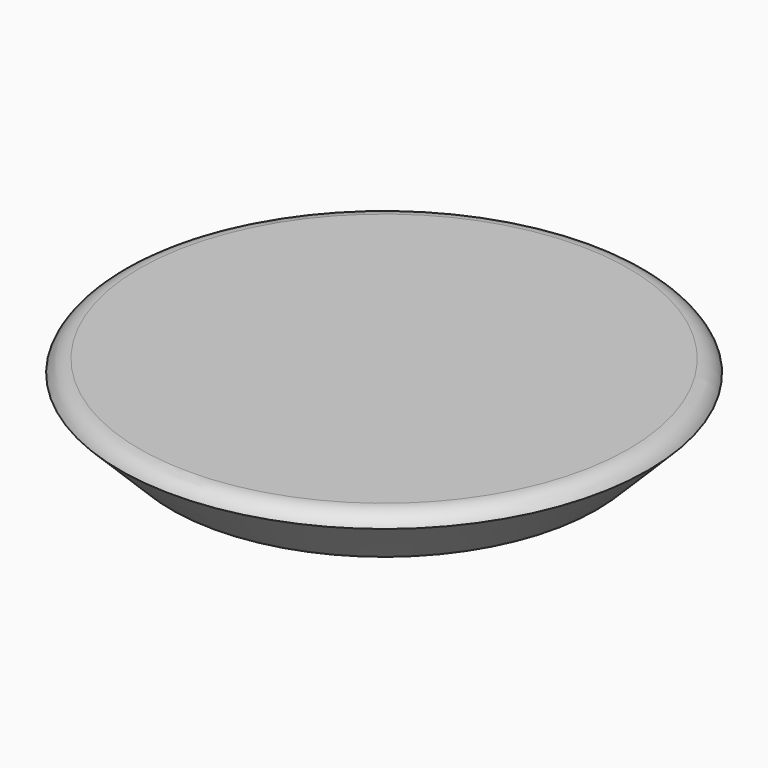
from build123d import *

# Parameters (mm, degrees)
F0_R     = 25
F1_DEPTH = 3
F2_R     = 2


# Not quite as in the source:
# - a fillet or chamfer that OpenCascade refuses, or shapes differently, is made with other operations: its cross-section is extruded or revolved along the edge and cut away or added


with BuildPart() as f1:
    # F0 (on Top) → F1 (new body, symmetric)
    with BuildSketch(Plane.XY):
        Circle(F0_R)
    extrude(amount=F1_DEPTH, both=True)

    # F2
    f2_edges = [f1.edges().sort_by_distance(p)[0] for p in [
        (-25, 0, 3),
    ]]
    fillet(f2_edges, radius=F2_R)

    # F3: chamfer of 5 on 1 edges, made by hand

    # F3_s1 → F3_t2 (revolve, cut)
    with BuildSketch(Plane.XZ):
        Polygon((25, 2), (20, -3), (25, -3), align=None)
    revolve(axis=Axis((0, 0, -3), (0, 0, 1)), mode=Mode.SUBTRACT)


solid = f1.part
